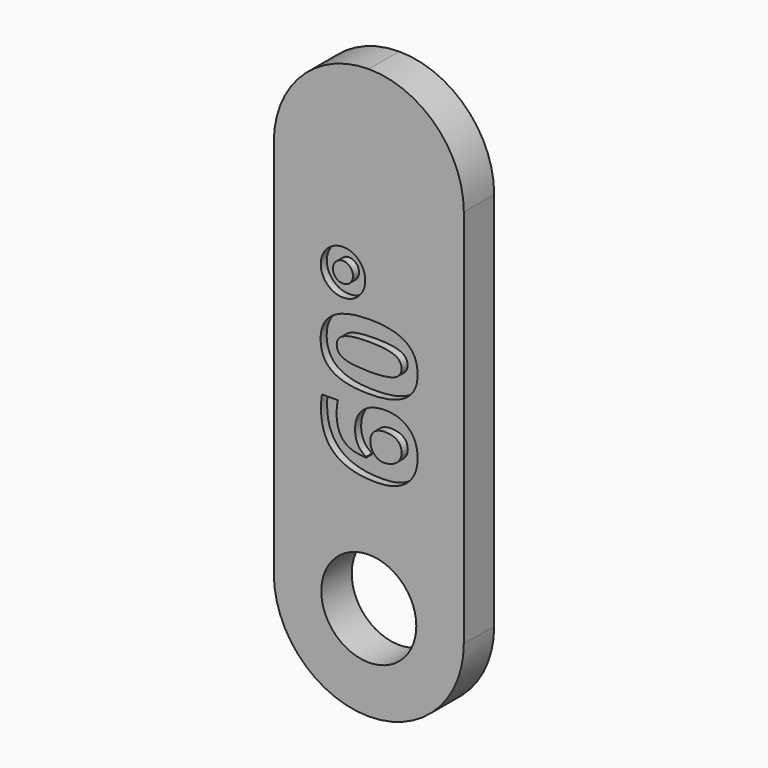
from build123d import *

# Parameters (mm, degrees)
F0_W         = 12.7
F0_H         = 38.1
F0_R         = 3.175
F1_DEPTH     = 2.54
F2_R         = 6.34999
F3_TEXT_SIZE = 8.8194444444
F4_DEPTH     = 0.508


# Not quite as in the source:
# - a fillet or chamfer is up to 0.001 mm smaller than in the source, because OpenCascade refuses the exact size
# - Text() gives the source's letters only with a copy of the font that has no kerning and outlines rounded to 1/6400 em; it was checked with that copy


with BuildPart() as f1:
    # F0 (on Front) → F1 (new body)
    with BuildSketch(Plane.XZ):
        with Locations((6.35, 19.05)):
            Rectangle(F0_W, F0_H)
        with Locations((6.35, 6.35)):
            Circle(F0_R, mode=Mode.SUBTRACT)
    extrude(amount=F1_DEPTH)

    # F2 (radius 6.35 in the source; OpenCascade refuses exactly that, so slightly less here)
    f2_edges = [f1.edges().sort_by_distance(p)[0] for p in [
        (12.7, -1.27, 0),
        (0, -1.27, 0),
        (12.7, -1.27, 38.1),
        (0, -1.27, 38.1),
    ]]
    fillet(f2_edges, radius=F2_R)

    # F3 (on face) → F4 (cut)
    with BuildSketch(Plane.XZ.offset(2.54)):
        with Locations(Location((9.525, 13.6294867622), (0, 0, 90))):
            Text('60°', F3_TEXT_SIZE, font='Open Sans', font_style=FontStyle.BOLD, text_align=(TextAlign.LEFT, TextAlign.BOTTOM))
    extrude(amount=-F4_DEPTH, mode=Mode.SUBTRACT)


solid = f1.part
